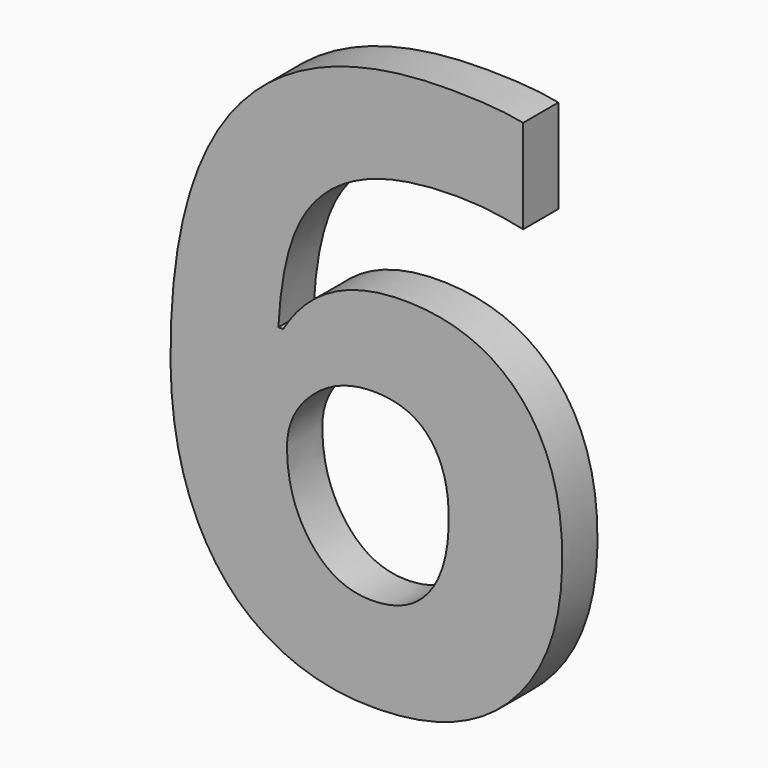
from build123d import *

# Parameters (mm, degrees)
F0_TEXT_SIZE = 70.5555555556
F1_DEPTH     = 4


# Not quite as in the source:
# - Text() gives the source's letters only with a copy of the font that has no kerning and outlines rounded to 1/6400 em; it was checked with that copy


with BuildPart() as f1:
    # F0 (on Front) → F1 (new body)
    with BuildSketch(Plane.XZ):
        with Locations((0, 0)):
            Text('6', F0_TEXT_SIZE, font='Open Sans', font_style=FontStyle.BOLD, text_align=(TextAlign.LEFT, TextAlign.BOTTOM))
    extrude(amount=F1_DEPTH)


solid = f1.part
